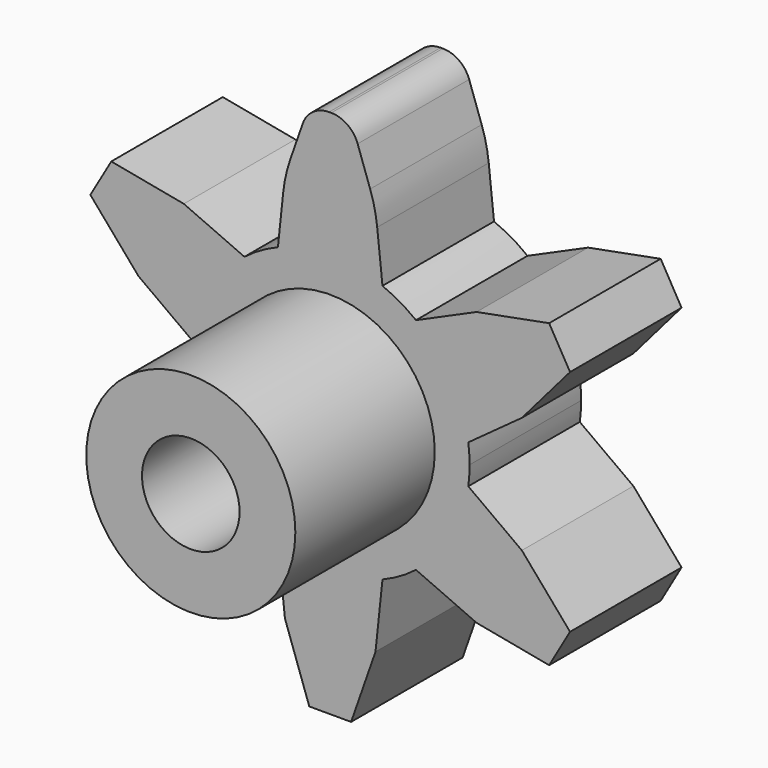
from build123d import *

# Parameters (mm, degrees)
F0_R     = 1.778
F1_DEPTH = 5.08
F2_R     = 3.81
F2_R_2   = 1.778
F3_DEPTH = 6.35
F4_R     = 5.08
F5_R     = 1.016


# Not quite as in the source:
# - a feature names something its author has since deleted; it is built from what else it names


with BuildPart() as f1:
    # F0 (on Front) → F1 (new body)
    with BuildSketch(Plane.XZ):
        with BuildLine():
            ThreePointArc((5.0308613437, -0.7048646254), (5.0677004463, -0.353287683), (5.08, 0))
            ThreePointArc((5.08, 0), (5.0677004463, 0.353287683), (5.0308613437, 0.7048646254))
            ThreePointArc((5.0308613437, 0.7048646254), (4.3994090512, 2.54), (3.1258613437, 4.0044214139))
            ThreePointArc((3.1258613437, 4.0044214139), (2.54, 4.3994090512), (1.905, 4.7092860393))
            ThreePointArc((1.905, 4.7092860393), (0, 5.08), (-1.905, 4.7092860393))
            ThreePointArc((-1.905, 4.7092860393), (-2.54, 4.3994090512), (-3.1258613437, 4.0044214139))
            ThreePointArc((-3.1258613437, 4.0044214139), (-4.3994090512, 2.54), (-5.0308613437, 0.7048646254))
            ThreePointArc((-5.0308613437, 0.7048646254), (-5.08, 0), (-5.0308613437, -0.7048646254))
            ThreePointArc((-5.0308613437, -0.7048646254), (-4.3994090512, -2.54), (-3.1258613437, -4.0044214139))
            ThreePointArc((-3.1258613437, -4.0044214139), (-2.54, -4.3994090512), (-1.905, -4.7092860393))
            ThreePointArc((-1.905, -4.7092860393), (0, -5.08), (1.905, -4.7092860393))
            ThreePointArc((1.905, -4.7092860393), (2.54, -4.3994090512), (3.1258613437, -4.0044214139))
            ThreePointArc((3.1258613437, -4.0044214139), (4.3994090512, -2.54), (5.0308613437, -0.7048646254))
        make_face()
        Circle(F0_R, mode=Mode.SUBTRACT)
        with BuildLine():
            ThreePointArc((3.1258613437, 4.0044214139), (4.3994090512, 2.54), (5.0308613437, 0.7048646254))
            Line((5.0308613437, 0.7048646254), (6.9846726717, 2.1261920584))
            Line((6.9846726717, 2.1261920584), (8.7398771973, 4.1660886423))
            Line((8.7398771973, 4.1660886423), (7.9778771973, 5.4859113577))
            Line((7.9778771973, 5.4859113577), (5.3336726717, 4.9858079416))
            Line((5.3336726717, 4.9858079416), (3.1258613437, 4.0044214139))
        make_face()
        with BuildLine():
            Line((6.9846726717, -2.1261920584), (5.0308613437, -0.7048646254))
            ThreePointArc((5.0308613437, -0.7048646254), (4.3994090512, -2.54), (3.1258613437, -4.0044214139))
            Line((3.1258613437, -4.0044214139), (5.3336726717, -4.9858079416))
            Line((5.3336726717, -4.9858079416), (7.9778771973, -5.4859113577))
            Line((7.9778771973, -5.4859113577), (8.7398771973, -4.1660886423))
            Line((8.7398771973, -4.1660886423), (6.9846726717, -2.1261920584))
        make_face()
        with BuildLine():
            ThreePointArc((-1.905, 4.7092860393), (0, 5.08), (1.905, 4.7092860393))
            Line((1.905, 4.7092860393), (1.651, 7.112))
            Line((1.651, 7.112), (0.762, 9.652))
            Line((0.762, 9.652), (-0.762, 9.652))
            Line((-0.762, 9.652), (-1.651, 7.112))
            Line((-1.651, 7.112), (-1.905, 4.7092860393))
        make_face()
        with BuildLine():
            Line((1.651, -7.112), (1.905, -4.7092860393))
            ThreePointArc((1.905, -4.7092860393), (0, -5.08), (-1.905, -4.7092860393))
            Line((-1.905, -4.7092860393), (-1.651, -7.112))
            Line((-1.651, -7.112), (-0.762, -9.652))
            Line((-0.762, -9.652), (0.762, -9.652))
            Line((0.762, -9.652), (1.651, -7.112))
        make_face()
        with BuildLine():
            ThreePointArc((-5.0308613437, 0.7048646254), (-4.3994090512, 2.54), (-3.1258613437, 4.0044214139))
            Line((-3.1258613437, 4.0044214139), (-5.3336726717, 4.9858079416))
            Line((-5.3336726717, 4.9858079416), (-7.9778771973, 5.4859113577))
            Line((-7.9778771973, 5.4859113577), (-8.7398771973, 4.1660886423))
            Line((-8.7398771973, 4.1660886423), (-6.9846726717, 2.1261920584))
            Line((-6.9846726717, 2.1261920584), (-5.0308613437, 0.7048646254))
        make_face()
        with BuildLine():
            Line((-5.3336726717, -4.9858079416), (-3.1258613437, -4.0044214139))
            ThreePointArc((-3.1258613437, -4.0044214139), (-4.3994090512, -2.54), (-5.0308613437, -0.7048646254))
            Line((-5.0308613437, -0.7048646254), (-6.9846726717, -2.1261920584))
            Line((-6.9846726717, -2.1261920584), (-8.7398771973, -4.1660886423))
            Line((-8.7398771973, -4.1660886423), (-7.9778771973, -5.4859113577))
            Line((-7.9778771973, -5.4859113577), (-5.3336726717, -4.9858079416))
        make_face()
    extrude(amount=F1_DEPTH)

    # F2 (on face) → F3 (join)
    with BuildSketch(Plane.XZ.offset(5.08)):
        Circle(F2_R)
        Circle(F2_R_2, mode=Mode.SUBTRACT)
    extrude(amount=F3_DEPTH)

    # F4
    f4_edges = [f1.edges().sort_by_distance(p)[0] for p in [
        (1.651, -2.54, 7.112),
        (-1.651, -2.54, 7.112),
    ]]
    fillet(f4_edges, radius=F4_R)

    # F5
    f5_edges = [f1.edges().sort_by_distance(p)[0] for p in [
        (0.762, -2.54, 9.652),
        (-0.762, -2.54, 9.652),
    ]]
    fillet(f5_edges, radius=F5_R)


solid = f1.part
